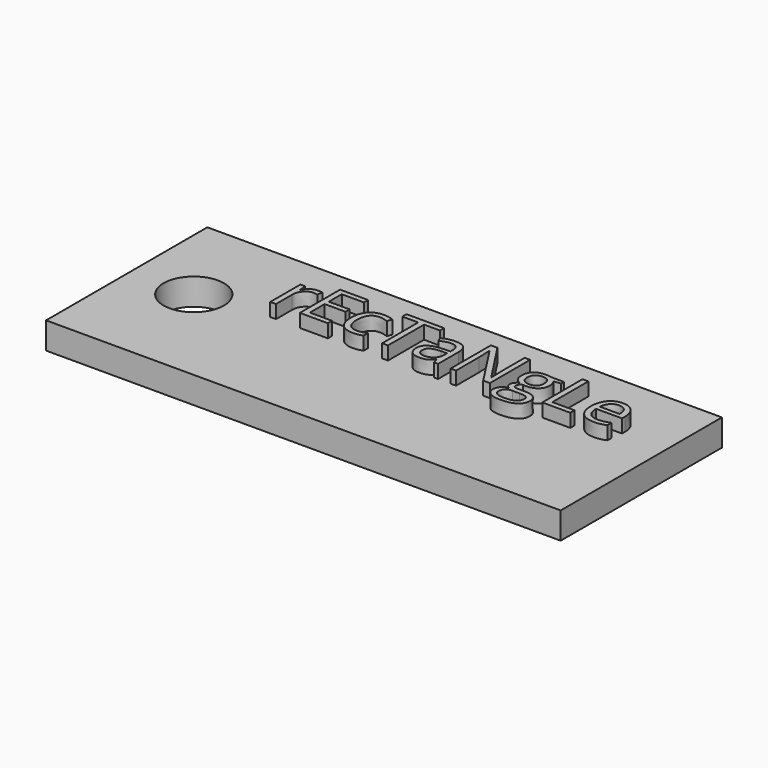
from build123d import *

# Parameters (mm, degrees)
F0_W         = 98.0302281678
F0_H         = 38.3920669556
F1_DEPTH     = 5.08
F2_R         = 5.7536432188
F3_DEPTH     = 25.4
F4_TEXT_SIZE = 13.4123076364
F5_DEPTH     = 2.54


# Not quite as in the source:
# - Text() gives the source's letters only with a copy of the font that has no kerning and outlines rounded to 1/6400 em; it was checked with that copy


with BuildPart() as f1:
    # F0 (on Top) → F1 (new body)
    with BuildSketch(Plane.XY):
        with Locations((-1.3983193785, -1.0647568852)):
            Rectangle(F0_W, F0_H)
    extrude(amount=F1_DEPTH)

    # F2 (on face) → F3 (cut)
    with BuildSketch(Plane.XY.offset(5.08)):
        with Locations((-38.4857989848, 0)):
            Circle(F2_R)
    extrude(amount=-F3_DEPTH, mode=Mode.SUBTRACT)

    # F4 (on face) → F5 (join)
    with BuildSketch(Plane.XY.offset(5.08)):
        with Locations((-26.1854305863, 1.3923830546)):
            Text('rEcTaNgLe', F4_TEXT_SIZE, font='Open Sans', text_align=(TextAlign.LEFT, TextAlign.BOTTOM))
    extrude(amount=F5_DEPTH)


solid = f1.part
